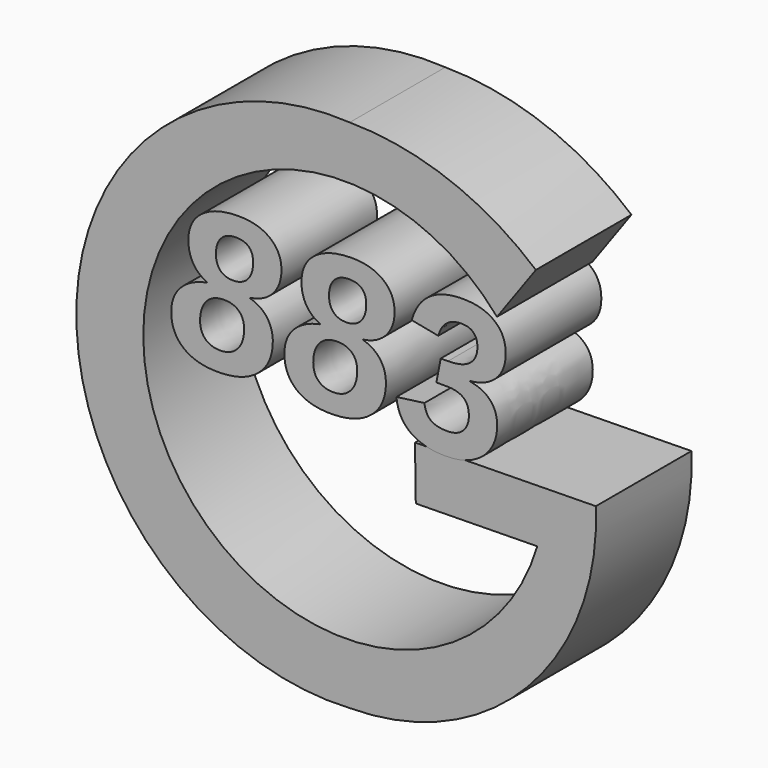
from build123d import *

# Parameters (mm, degrees)
F2_DEPTH     = 25.4
F1_TEXT_SIZE = 43.2398383661
F3_DEPTH     = 25.4


# Not quite as in the source:
# - Text() gives the source's letters only with a copy of the font that has no kerning and outlines rounded to 1/6400 em; it was checked with that copy


with BuildPart() as f2:
    # F0 (on Front) → F2 (new body)
    with BuildSketch(Plane.XZ):
        with BuildLine():
            ThreePointArc((39.5680703223, 40.6490378082), (21.0941177868, 51.5335496506), (0, 55.3803294897))
            ThreePointArc((0, 55.3803294897), (-58.1191567909, 0.5829520524), (0, -54.214425385))
            ThreePointArc((0, -54.214425385), (37.8070387991, -37.9361986755), (52.3200631142, 0.5829520524))
            Line((52.3200631142, 0.5829520524), (13.8720208779, 0))
            Line((13.8720208779, 0), (14.0443156626, -11.3635369017))
            Line((14.0443156626, -11.3635369017), (39.8704148829, -10.9719596803))
            ThreePointArc((39.8704148829, -10.9719596803), (-42.9454646375, -7.6387077748), (31.306155026, 29.1889645159))
            Line((31.306155026, 29.1889645159), (39.5680703223, 40.6490378082))
        make_face()
    extrude(amount=F2_DEPTH)


with BuildPart() as f3:
    # F1 (on Front) → F3 (new body)
    with BuildSketch(Plane.XZ):
        with Locations((-38.4952125581, 0)):
            Text('883', F1_TEXT_SIZE, font='Arimo', font_style=FontStyle.BOLDITALIC, text_align=(TextAlign.LEFT, TextAlign.BOTTOM))
    extrude(amount=F3_DEPTH)


solid = Compound([f2.part, f3.part])
